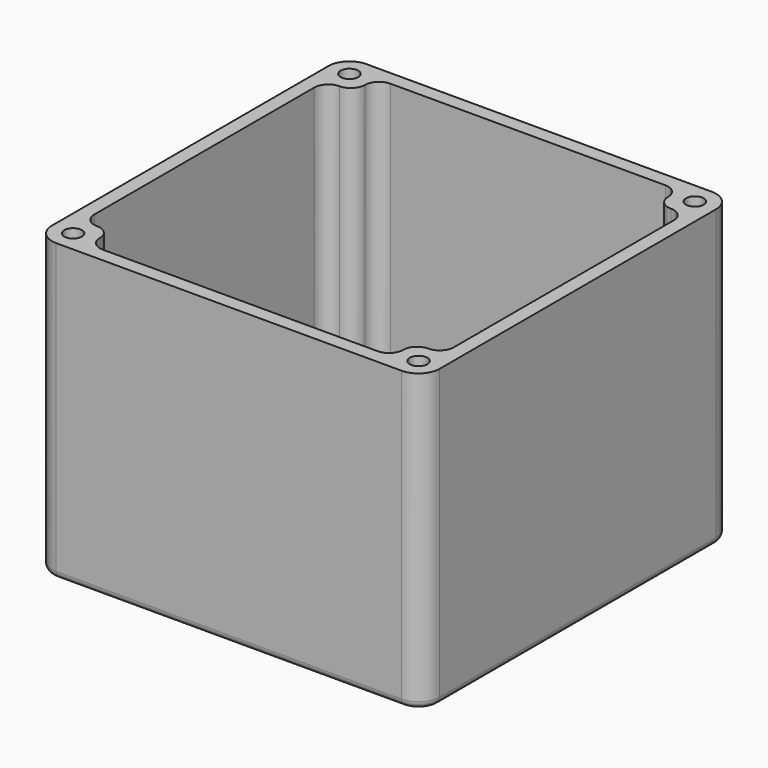
from build123d import *

# Parameters (mm, degrees)
F0_W     = 55
F0_H     = 55
F0_R     = 1.5
F0_R_2   = 18.75
F1_DEPTH = 2
F2_W     = 55
F2_H     = 55
F3_DEPTH = 40
F4_R     = 1.25
F5_DEPTH = 10
F6_R     = 3
F7_R     = 1
F8_F1_R  = 2
F8_F2_R  = 1.9999


# Not quite as in the source:
# - a fillet or chamfer is up to 0.001 mm smaller than in the source, because OpenCascade refuses the exact size


with BuildPart() as f1:
    # F0 (on Top) → F1 (new body)
    with BuildSketch(Plane.XY):
        Rectangle(F0_W, F0_H)
        with Locations((-16.65, -16.65)):
            Circle(F0_R, mode=Mode.SUBTRACT)
        with Locations((16.65, -16.65)):
            Circle(F0_R, mode=Mode.SUBTRACT)
        with Locations((-16.65, 16.65)):
            Circle(F0_R, mode=Mode.SUBTRACT)
        with Locations((0, 0.5)):
            Circle(F0_R_2, mode=Mode.SUBTRACT)
        with Locations((16.65, 16.65)):
            Circle(F0_R, mode=Mode.SUBTRACT)
    extrude(amount=F1_DEPTH)

    # F2 (on face) → F3 (join)
    with BuildSketch(Plane.XY.offset(2)):
        Rectangle(F2_W, F2_H)
        Polygon((-21.5, 21.5), (-21.5, 25.5), (21.5, 25.5), (21.5, 21.5), (25.5, 21.5), (25.5, -21.5), (21.5, -21.5), (21.5, -25.5), (-21.5, -25.5), (-21.5, -21.5), (-25.5, -21.5), (-25.5, 21.5), align=None, mode=Mode.SUBTRACT)
    extrude(amount=F3_DEPTH)

    # F4 (on face) → F5 (cut)
    with BuildSketch(Plane.XY.offset(42)):
        with Locations((-24.5, 24.5)):
            Circle(F4_R)
        with Locations((-24.5, -24.5)):
            Circle(F4_R)
        with Locations((24.5, -24.5)):
            Circle(F4_R)
        with Locations((24.5, 24.5)):
            Circle(F4_R)
    extrude(amount=-F5_DEPTH, mode=Mode.SUBTRACT)

    # F6
    f6_edges = [f1.edges().sort_by_distance(p)[0] for p in [
        (-27.5, -27.5, 21),
        (27.5, -27.5, 21),
        (-27.5, 27.5, 21),
        (27.5, 27.5, 21),
    ]]
    fillet(f6_edges, radius=F6_R)

    # F7
    f7_edges = [f1.edges().sort_by_distance(p)[0] for p in [
        (0, -27.5, 0),
        (27.5, 0, 0),
        (26.62132, -26.62132, 0),
        (26.62132, 26.62132, 0),
        (0, 27.5, 0),
        (-26.62132, -26.62132, 0),
        (-26.62132, 26.62132, 0),
        (-27.5, 0, 0),
    ]]
    fillet(f7_edges, radius=F7_R)

    # F8: fillet of radius 2 on 20 edges, made by hand

    # F8_f1
    f8_f1_edges = [f1.edges().sort_by_distance(p)[0] for p in [
        (21.5, -21.5, 22),
        (-21.5, -21.5, 22),
        (-21.5, 21.5, 22),
        (21.5, 21.5, 22),
    ]]
    fillet(f8_f1_edges, radius=F8_F1_R)

    # F8_f2 (radius 2 in the source; OpenCascade refuses exactly that, so slightly less here)
    f8_f2_edges = [f1.edges().sort_by_distance(p)[0] for p in [
        (-21.5, -25.5, 22),
        (-25.5, -21.5, 22),
        (21.5, -25.5, 22),
        (25.5, -21.5, 22),
        (-25.5, 21.5, 22),
        (-21.5, 25.5, 22),
        (21.5, 25.5, 22),
        (25.5, 21.5, 22),
        (0, -25.5, 2),
        (25.5, 0, 2),
        (-25.5, 0, 2),
        (0, 25.5, 2),
        (-24.5, -21.5, 2),
        (-21.5, 24.5, 2),
        (21.5, -24.5, 2),
        (24.5, 21.5, 2),
        (22.0857864376, 22.0857864376, 2),
        (22.0857864376, -22.0857864376, 2),
        (-22.0857864376, 22.0857864376, 2),
        (-22.0857864376, -22.0857864376, 2),
    ]]
    fillet(f8_f2_edges, radius=F8_F2_R)


solid = f1.part
